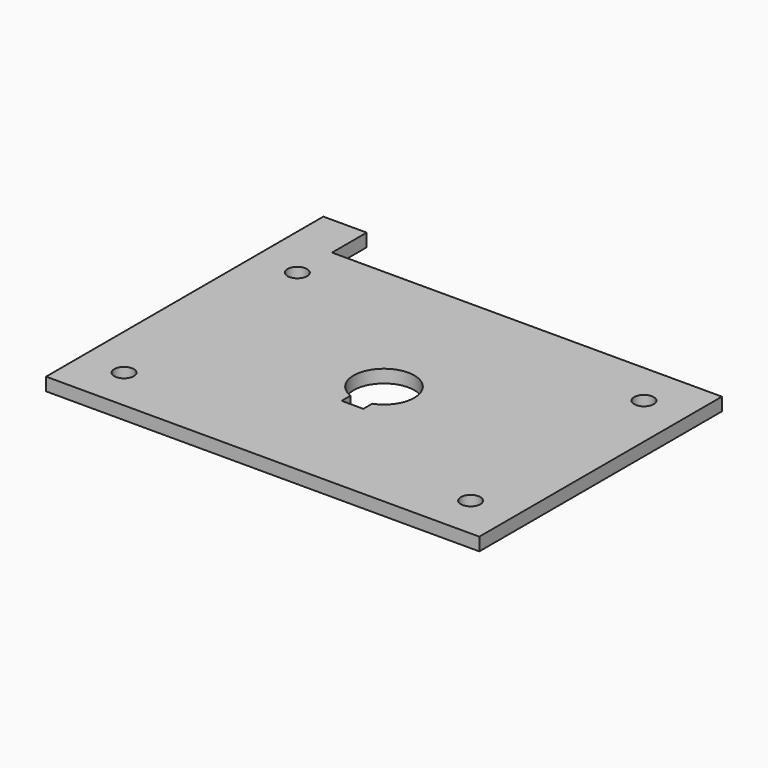
from build123d import *

# Parameters (mm, degrees)
F0_R     = 2.25
F0_W     = 10
F0_H     = 10
F1_DEPTH = 3


# Not quite as in the source:
# - a feature names something its author has since deleted; it is built from what else it names


with BuildPart() as f1:
    # F0 (on Top) → F1 (new body)
    with BuildSketch(Plane.XY):
        Polygon((-50, -40.0267248601), (50, -40.0267248601), (50, 29.9732751399), (-40, 29.9732751399), (-50, 29.9732751399), align=None)
        with Locations((-40, -30.0267248601)):
            Circle(F0_R, mode=Mode.SUBTRACT)
        with Locations((40, -30.0267248601)):
            Circle(F0_R, mode=Mode.SUBTRACT)
        with BuildLine():
            Line((-2.5, -14.1267248601), (-2.5, -11.5650732754))
            ThreePointArc((-2.5, -11.5650732754), (-3.9686269666, 0.7395564373), (7, -5.0267248601))
            ThreePointArc((7, -5.0267248601), (5.7662812973, -8.9953518267), (2.5, -11.5650732754))
            Line((2.5, -11.5650732754), (2.5, -14.1267248601))
            Line((2.5, -14.1267248601), (-2.5, -14.1267248601))
        make_face(mode=Mode.SUBTRACT)
        with Locations((-40, 19.9732751399)):
            Circle(F0_R, mode=Mode.SUBTRACT)
        with Locations((40, 19.9732751399)):
            Circle(F0_R, mode=Mode.SUBTRACT)
        with Locations((-45, 34.9732751399)):
            Rectangle(F0_W, F0_H)
    extrude(amount=F1_DEPTH)


solid = f1.part
